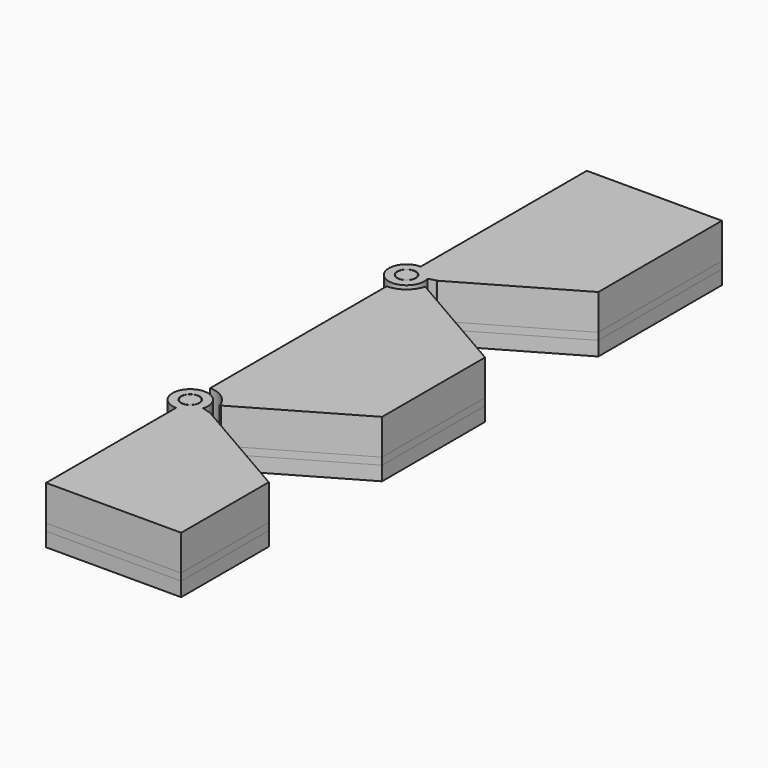
from build123d import *

# Parameters (mm, degrees)
F1_DEPTH = 2
F0_R     = 2.5
F3_DEPTH = 1
F2_R     = 1.25
F4_R     = 1.3
F5_DEPTH = 5
F4_R_2   = 1.25


# Not quite as in the source:
# - a feature of the source that left no trace in its solid (it failed there, or was rolled back) is left out


with BuildPart() as f1:
    # F0 (on Top) → F1 (new body)
    with BuildSketch(Plane.XY):
        with BuildLine():
            Line((0, 49.5557405042), (-19.05, 49.5557405042))
            Line((-19.05, 49.5557405042), (-19.05, 21.3057405042))
            ThreePointArc((-19.05, 21.3057405042), (-16.9583499337, 20.6119835443), (-15.6958980338, 18.8057405042))
            Line((-15.6958980338, 18.8057405042), (-15.55, 18.8057405042))
            Line((-15.55, 18.8057405042), (0, 27.7835371901))
            Line((0, 27.7835371901), (0, 49.5557405042))
        make_face()
    extrude(amount=F1_DEPTH)


with BuildPart() as f1b:
    # F0 (on Top) → F1, piece 2 (new body)
    with BuildSketch(Plane.XY):
        with BuildLine():
            Line((0, -10.3164628099), (0, 7.8279438183))
            Line((0, 7.8279438183), (-15.55, 16.8057405042))
            Line((-15.55, 16.8057405042), (-15.6958980338, 16.8057405042))
            ThreePointArc((-15.6958980338, 16.8057405042), (-16.9583499337, 14.9994974641), (-19.05, 14.3057405042))
            Line((-19.05, 14.3057405042), (-19.05, -16.7942594958))
            ThreePointArc((-19.05, -16.7942594958), (-16.9583499337, -17.4880164557), (-15.6958980338, -19.2942594958))
            Line((-15.6958980338, -19.2942594958), (-15.55, -19.2942594958))
            Line((-15.55, -19.2942594958), (0, -10.3164628099))
        make_face()
    extrude(amount=F1_DEPTH)


with BuildPart() as f1c:
    # F0 (on Top) → F1, piece 3 (new body)
    with BuildSketch(Plane.XY):
        with BuildLine():
            Line((-19.05, -23.7942594958), (-19.05, -45.6942594958))
            Line((-19.05, -45.6942594958), (-0.0095496495, -45.6942594958))
            Line((-0.0095496495, -45.6942594958), (-0.0095496495, -30.266542689))
            Line((-0.0095496495, -30.266542689), (-15.55, -21.2942594958))
            Line((-15.55, -21.2942594958), (-15.6958980338, -21.2942594958))
            ThreePointArc((-15.6958980338, -21.2942594958), (-16.9583499337, -23.1005025359), (-19.05, -23.7942594958))
        make_face()
    extrude(amount=F1_DEPTH)


with BuildPart() as f1d:
    # F0 (on Top) → F1, piece 4 (new body)
    with BuildSketch(Plane.XY):
        with Locations((-19.05, 17.8057405042)):
            Circle(F0_R)
    extrude(amount=F1_DEPTH)


with BuildPart() as f1e:
    # F0 (on Top) → F1, piece 5 (new body)
    with BuildSketch(Plane.XY):
        with Locations((-19.05, -20.2942594958)):
            Circle(F0_R)
    extrude(amount=F1_DEPTH)


with BuildPart() as f3:
    # F2 (on face) → F3 (new body)
    with BuildSketch(Plane.XY.offset(2)):
        with BuildLine():
            ThreePointArc((-19.05, 21.3057405042), (-16.9583499337, 20.6119835443), (-15.6958980338, 18.8057405042))
            Line((-15.6958980338, 18.8057405042), (-15.55, 18.8057405042))
            Line((-15.55, 18.8057405042), (0, 27.7835371901))
            Line((0, 27.7835371901), (0, 49.5557405042))
            Line((0, 49.5557405042), (-19.05, 49.5557405042))
            Line((-19.05, 49.5557405042), (-19.05, 21.3057405042))
        make_face()
    extrude(amount=F3_DEPTH)


with BuildPart() as f3b:
    # F2 (on face) → F3, piece 2 (new body)
    with BuildSketch(Plane.XY.offset(2)):
        with BuildLine():
            Line((-15.55, 16.8057405042), (-15.6958980338, 16.8057405042))
            ThreePointArc((-15.6958980338, 16.8057405042), (-16.9583499337, 14.9994974641), (-19.05, 14.3057405042))
            Line((-19.05, 14.3057405042), (-19.05, -16.7942594958))
            ThreePointArc((-19.05, -16.7942594958), (-16.9583499337, -17.4880164557), (-15.6958980338, -19.2942594958))
            Line((-15.6958980338, -19.2942594958), (-15.55, -19.2942594958))
            Line((-15.55, -19.2942594958), (0, -10.3164628099))
            Line((0, -10.3164628099), (0, 7.8279438183))
            Line((0, 7.8279438183), (-15.55, 16.8057405042))
        make_face()
    extrude(amount=F3_DEPTH)


with BuildPart() as f3c:
    # F2 (on face) → F3, piece 3 (new body)
    with BuildSketch(Plane.XY.offset(2)):
        with BuildLine():
            Line((-0.0095496495, -45.6942594958), (-0.0095496495, -30.266542689))
            Line((-0.0095496495, -30.266542689), (-15.55, -21.2942594958))
            Line((-15.55, -21.2942594958), (-15.6958980338, -21.2942594958))
            ThreePointArc((-15.6958980338, -21.2942594958), (-16.9583499337, -23.1005025359), (-19.05, -23.7942594958))
            Line((-19.05, -23.7942594958), (-19.05, -45.6942594958))
            Line((-19.05, -45.6942594958), (-0.0095496495, -45.6942594958))
        make_face()
    extrude(amount=F3_DEPTH)


with BuildPart() as f3d:
    # F2 (on face) → F3, piece 4 (new body)
    with BuildSketch(Plane.XY.offset(2)):
        with Locations((-19.05, 17.8057405042)):
            Circle(F2_R)
    extrude(amount=F3_DEPTH)


with BuildPart() as f3e:
    # F2 (on face) → F3, piece 5 (new body)
    with BuildSketch(Plane.XY.offset(2)):
        with Locations((-19.05, -20.2942594958)):
            Circle(F2_R)
    extrude(amount=F3_DEPTH)


with BuildPart() as f5:
    # F4 (on face) → F5 (new body)
    with BuildSketch(Plane.XY.offset(3)):
        with BuildLine():
            Line((-16.6542128813, 18.5200262185), (-15.6958980338, 18.8057405042))
            Line((-15.6958980338, 18.8057405042), (-15.55, 18.8057405042))
            Line((-15.55, 18.8057405042), (0, 27.7835371901))
            Line((0, 27.7835371901), (0, 49.5557405042))
            Line((0, 49.5557405042), (-19.05, 49.5557405042))
            Line((-19.05, 49.5557405042), (-19.05, 21.3057405042))
            Line((-19.05, 21.3057405042), (-19.05, 20.3057405042))
            ThreePointArc((-19.05, 20.3057405042), (-20.5440357617, 15.8012811898), (-16.6542128813, 18.5200262185))
        make_face()
        with Locations((-19.05, 17.8057405042)):
            Circle(F4_R, mode=Mode.SUBTRACT)
    extrude(amount=F5_DEPTH)


with BuildPart() as f5b:
    # F4 (on face) → F5, piece 2 (new body)
    with BuildSketch(Plane.XY.offset(3)):
        with BuildLine():
            Line((0, -10.3164628099), (0, 7.8279438183))
            Line((0, 7.8279438183), (-15.55, 16.8057405042))
            Line((-15.55, 16.8057405042), (-15.6958980338, 16.8057405042))
            ThreePointArc((-15.6958980338, 16.8057405042), (-16.9583499337, 14.9994974641), (-19.05, 14.3057405042))
            Line((-19.05, 14.3057405042), (-19.05, -16.7942594958))
            ThreePointArc((-19.05, -16.7942594958), (-16.9583499337, -17.4880164557), (-15.6958980338, -19.2942594958))
            Line((-15.6958980338, -19.2942594958), (-15.55, -19.2942594958))
            Line((-15.55, -19.2942594958), (0, -10.3164628099))
        make_face()
    extrude(amount=F5_DEPTH)


with BuildPart() as f5c:
    # F4 (on face) → F5, piece 3 (new body)
    with BuildSketch(Plane.XY.offset(3)):
        with BuildLine():
            Line((-19.05, -23.7942594958), (-19.05, -45.6942594958))
            Line((-19.05, -45.6942594958), (-0.0095496495, -45.6942594958))
            Line((-0.0095496495, -45.6942594958), (-0.0095496495, -30.266542689))
            Line((-0.0095496495, -30.266542689), (-15.55, -21.2942594958))
            Line((-15.55, -21.2942594958), (-15.6958980338, -21.2942594958))
            Line((-15.6958980338, -21.2942594958), (-16.6542128813, -21.0085452101))
            ThreePointArc((-16.6542128813, -21.0085452101), (-20.5440357617, -18.2898001815), (-19.05, -22.7942594958))
            Line((-19.05, -22.7942594958), (-19.05, -23.7942594958))
        make_face()
        with Locations((-19.05, -20.2942594958)):
            Circle(F4_R, mode=Mode.SUBTRACT)
    extrude(amount=F5_DEPTH)


with BuildPart() as f5d:
    # F4 (on face) → F5, piece 4 (new body)
    with BuildSketch(Plane.XY.offset(3)):
        with Locations((-19.05, 17.8057405042)):
            Circle(F4_R_2)
    extrude(amount=F5_DEPTH)


with BuildPart() as f5e:
    # F4 (on face) → F5, piece 5 (new body)
    with BuildSketch(Plane.XY.offset(3)):
        with Locations((-19.05, -20.2942594958)):
            Circle(F4_R_2)
    extrude(amount=F5_DEPTH)


solid = Compound([f1.part, f1b.part, f1c.part, f1d.part, f1e.part, f3.part, f3b.part, f3c.part, f3d.part, f3e.part, f5.part, f5b.part, f5c.part, f5d.part, f5e.part])
